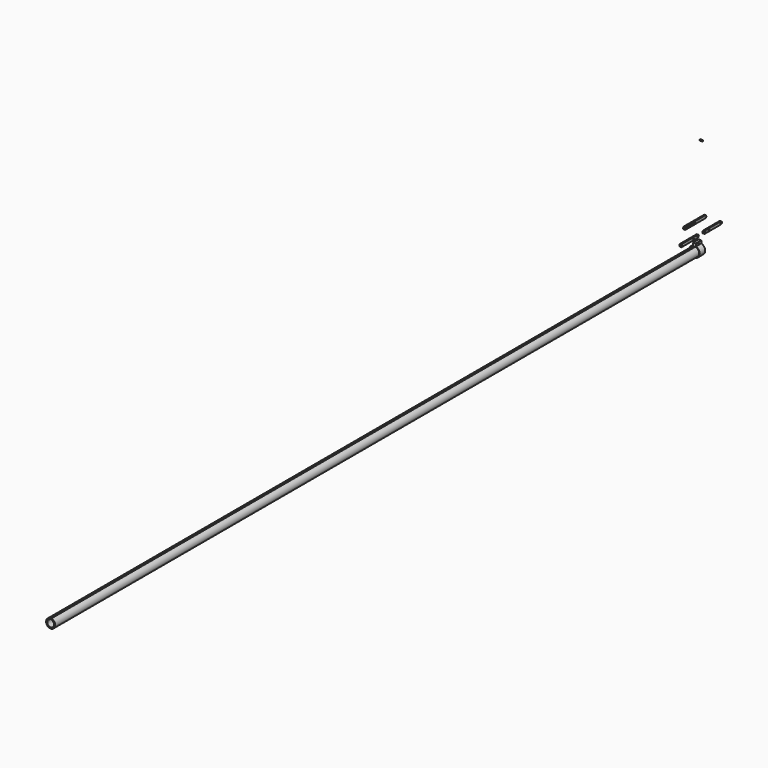
from build123d import *

# Parameters (mm, degrees)
F0_W          = 8.516
F0_H          = 1.016
F0_R          = 0.254
F1_DEPTH      = 0.508
F0_W_2        = 10.287
F2_R          = 0.50799
F2_2_R        = 0.50799
F2_3_R        = 0.50799
F4_DEPTH      = 304.8
F6_DEPTH      = 2.54
F7_R          = 0.254
F8_DEPTH      = 1.9695
F8_DEPTH_BACK = 1.9695
F9_R          = 0.2286
F10_DEPTH     = 1.016


# Not quite as in the source:
# - a fillet or chamfer is up to 0.001 mm smaller than in the source, because OpenCascade refuses the exact size


with BuildPart() as f1:
    # F0 (on Right) → F1 (new body)
    with BuildSketch(Plane.YZ):
        with Locations((-5.428305112, 4.8920463305)):
            Rectangle(F0_W, F0_H)
        with Locations((-9.178305112, 4.8920463305)):
            Circle(F0_R, mode=Mode.SUBTRACT)
        with Locations((-3.710305112, 4.8920463305)):
            Circle(F0_R, mode=Mode.SUBTRACT)
        with Locations((-1.678305112, 4.8920463305)):
            Circle(F0_R, mode=Mode.SUBTRACT)
    extrude(amount=F1_DEPTH)

    # F2#3 (radius 0.508 in the source; OpenCascade refuses exactly that, so slightly less here)
    f2_3_edges = [f1.edges().sort_by_distance(p)[0] for p in [
        (0.254, -1.170305, 5.400046),
        (0.254, -1.170305, 4.384046),
        (0.254, -9.686305, 5.400046),
        (0.254, -9.686305, 4.384046),
    ]]
    fillet(f2_3_edges, radius=F2_3_R)


with BuildPart() as f1b:
    # F0 (on Right) → F1, piece 2 (new body)
    with BuildSketch(Plane.YZ):
        with Locations((5.428305112, 4.8920463305)):
            Rectangle(F0_W, F0_H)
        with Locations((1.678305112, 4.8920463305)):
            Circle(F0_R, mode=Mode.SUBTRACT)
        with Locations((3.710305112, 4.8920463305)):
            Circle(F0_R, mode=Mode.SUBTRACT)
        with Locations((9.178305112, 4.8920463305)):
            Circle(F0_R, mode=Mode.SUBTRACT)
    extrude(amount=F1_DEPTH)

    # F2#2 (radius 0.508 in the source; OpenCascade refuses exactly that, so slightly less here)
    f2_2_edges = [f1b.edges().sort_by_distance(p)[0] for p in [
        (0.254, 9.686305, 5.400046),
        (0.254, 9.686305, 4.384046),
        (0.254, 1.170305, 5.400046),
        (0.254, 1.170305, 4.384046),
    ]]
    fillet(f2_2_edges, radius=F2_2_R)


with BuildPart() as f1c:
    # F0 (on Right) → F1, piece 3 (new body)
    with BuildSketch(Plane.YZ):
        with Locations((-2.7879898956, 9.9034412917)):
            Rectangle(F0_W_2, F0_H)
        with Locations((-7.4234898956, 9.9034412917)):
            Circle(F0_R, mode=Mode.SUBTRACT)
        with BuildLine():
            ThreePointArc((-6.4074898956, 9.9034412917), (-6.333095018, 10.0830464142), (-6.1534898956, 10.1574412917))
            Line((-6.1534898956, 10.1574412917), (-2.9784898956, 10.1574412917))
            ThreePointArc((-2.9784898956, 10.1574412917), (-2.7988847732, 10.0830464142), (-2.7244898956, 9.9034412917))
            ThreePointArc((-2.7244898956, 9.9034412917), (-2.7988847732, 9.7238361693), (-2.9784898956, 9.6494412917))
            Line((-2.9784898956, 9.6494412917), (-6.1534898956, 9.6494412917))
            ThreePointArc((-6.1534898956, 9.6494412917), (-6.333095018, 9.7238361693), (-6.4074898956, 9.9034412917))
        make_face(mode=Mode.SUBTRACT)
    extrude(amount=F1_DEPTH)

    # F2 (radius 0.508 in the source; OpenCascade refuses exactly that, so slightly less here)
    f2_edges = [f1c.edges().sort_by_distance(p)[0] for p in [
        (0.254, -7.93149, 10.411441),
        (0.254, -7.93149, 9.395441),
        (0.254, 2.35551, 10.411441),
        (0.254, 2.35551, 9.395441),
    ]]
    fillet(f2_edges, radius=F2_R)


with BuildPart() as f4:
    # F3 (on Front) → F4 (new body)
    with BuildSketch(Plane.XZ):
        with BuildLine():
            Line((-0.254, 1.2443407893), (-0.254, 1.6955808002))
            ThreePointArc((-0.254, 1.6955808002), (0, -1.7145), (0.254, 1.6955808002))
            Line((0.254, 1.6955808002), (0.254, 1.2443407893))
            ThreePointArc((0.254, 1.2443407893), (0, -1.27), (-0.254, 1.2443407893))
        make_face()
    extrude(amount=F4_DEPTH)


with BuildPart() as f6:
    # F5 (on Front) → F6 (new body)
    with BuildSketch(Plane.XZ):
        with BuildLine():
            Line((-0.508, 2.9178223497), (-0.508, 1.9018223497))
            ThreePointArc((-0.508, 1.9018223497), (0, -1.9685), (0.508, 1.9018223497))
            Line((0.508, 1.9018223497), (0.508, 2.9178223497))
            Line((0.508, 2.9178223497), (0, 2.9178223497))
            Line((0, 2.9178223497), (-0.508, 2.9178223497))
        make_face()
        with BuildLine():
            ThreePointArc((0.1905, 1.7677651852), (0, -1.778), (-0.1905, 1.7677651852))
            Line((-0.1905, 1.7677651852), (-0.1905, 1.27))
            Line((-0.1905, 1.27), (0.1905, 1.27))
            Line((0.1905, 1.27), (0.1905, 1.7677651852))
        make_face(mode=Mode.SUBTRACT)
    extrude(amount=F6_DEPTH)

    # F7 (on Right) → F8 (cut, two sides)
    with BuildSketch(Plane.YZ) as f8_sk:
        with Locations((-1.27, 2.4098223497)):
            Circle(F7_R)
    extrude(amount=-F8_DEPTH, mode=Mode.SUBTRACT)
    extrude(f8_sk.sketch, amount=F8_DEPTH_BACK, mode=Mode.SUBTRACT)


with BuildPart() as f10:
    # F9 (on Right) → F10 (new body)
    with BuildSketch(Plane.YZ):
        with Locations((0, 35.941991955)):
            Circle(F9_R)
    extrude(amount=F10_DEPTH)


solid = Compound([f1.part, f1b.part, f1c.part, f4.part, f6.part, f10.part])
